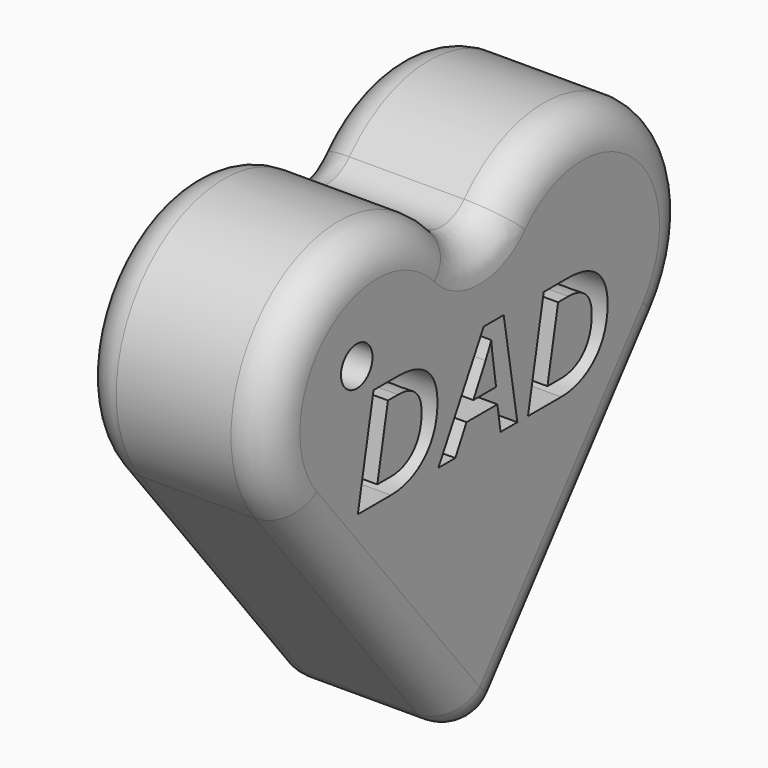
from build123d import *

# Parameters (mm, degrees)
F1_DEPTH     = 25.4
F2_TEXT_SIZE = 19.5592044731
F3_DEPTH     = 152.4
F4_F1_R      = 5.08
F4_F2_R      = 5.08
F5_R         = 2.6170235765
F6_DEPTH     = 152.4


# Not quite as in the source:
# - Text() gives the source's letters only with a copy of the font that has no kerning and outlines rounded to 1/6400 em; it was checked with that copy


with BuildPart() as f1:
    # F0 (on Right) → F1 (new body)
    with BuildSketch(Plane.YZ):
        with BuildLine():
            Line((-31.0266073793, 0), (0, -38.8684943318))
            Line((0, -38.8684943318), (31.0266073793, 0))
            ThreePointArc((31.0266073793, 0), (25.481787722, 26.9361923073), (0, 16.5929831564))
            ThreePointArc((0, 16.5929831564), (-25.481787722, 26.9361923073), (-31.0266073793, 0))
        make_face()
    extrude(amount=F1_DEPTH)

    # F2 (on face) → F3 (cut)
    with BuildSketch(Plane.YZ.offset(25.4)):
        with Locations((-20.5740000635, -2.2860001773)):
            Text('DAD', F2_TEXT_SIZE, font='Arimo', font_style=FontStyle.BOLDITALIC, text_align=(TextAlign.LEFT, TextAlign.BOTTOM))
    extrude(amount=-F3_DEPTH, mode=Mode.SUBTRACT)

    # F4: fillet of radius 5.08 on 5 edges, made by hand

    # F4_f1
    f4_f1_edges = [f1.edges().sort_by_distance(p)[0] for p in [
        (12.7, 0, 16.5929831564),
    ]]
    fillet(f4_f1_edges, radius=F4_F1_R)

    # F4_f2
    f4_f2_edges = [f1.edges().sort_by_distance(p)[0] for p in [
        (0, 28.6268169067, 24.7954921074),
        (25.4, 28.6268169067, 24.7954921074),
        (12.7, 0, -38.8684943318),
        (25.4, 15.5133036897, -19.4342471659),
        (0, 15.5133036897, -19.4342471659),
        (25.4, 0, 21.4779801589),
        (0, 0, 21.4779801589),
    ]]
    fillet(f4_f2_edges, radius=F4_F2_R)

    # F5 (on face) → F6 (cut)
    with BuildSketch(Plane.YZ.offset(25.4)):
        with Locations((-20.40335536, 15.1090240106)):
            Circle(F5_R)
    extrude(amount=-F6_DEPTH, mode=Mode.SUBTRACT)


solid = f1.part
